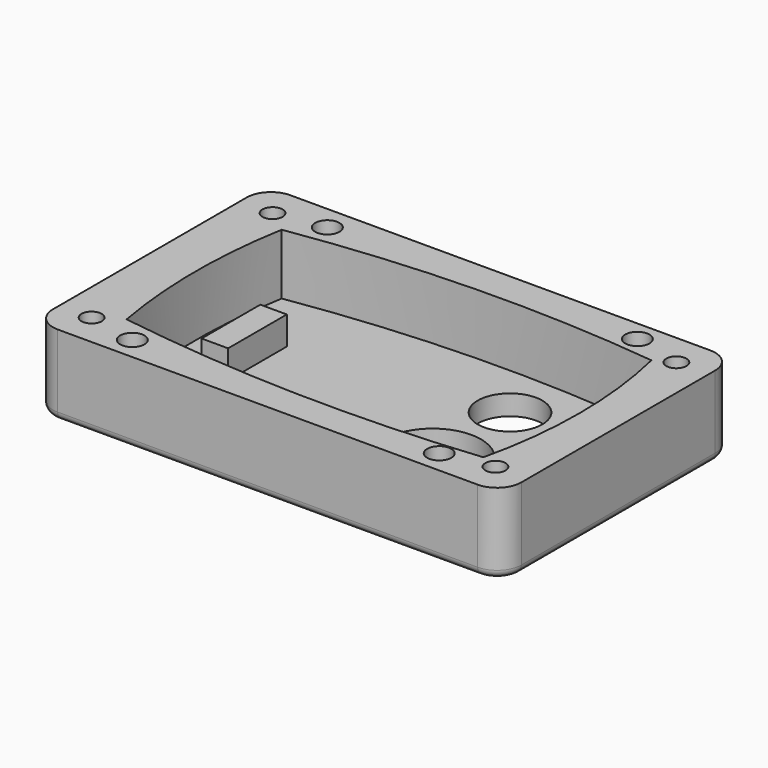
from build123d import *

# Parameters (mm, degrees)
F0_W     = 58
F0_H     = 36
F0_R     = 1.25
F0_R_2   = 1.5
F1_DEPTH = 10
F0_R_3   = 1
F0_W_2   = 3.2825097442
F0_H_2   = 9.0816104785
F0_R_4   = 4
F2_DEPTH = 2.5
F3_R     = 3
F4_DEPTH = 6
F5_START = 0.9
F5_DEPTH = 16.2
F6_START = 6
F6_DEPTH = 10.7
F7_R     = 1


with BuildPart() as f1:
    # F0 (on Top) → F1 (new body)
    with BuildSketch(Plane.XY):
        with Locations((22.1260370687, 12.181818096)):
            Rectangle(F0_W, F0_H)
        with Locations((-2.8739629313, -1.818181904)):
            Circle(F0_R, mode=Mode.SUBTRACT)
        with Locations((3.1260370687, -3.018181904)):
            Circle(F0_R_2, mode=Mode.SUBTRACT)
        with Locations((41.1260370687, -3.018181904)):
            Circle(F0_R_2, mode=Mode.SUBTRACT)
        with Locations((47.1260370687, -1.818181904)):
            Circle(F0_R, mode=Mode.SUBTRACT)
        with BuildLine():
            Line((-0.0042433119, 0.0237876128), (-0.0123524841, 0.02397218))
            Line((-0.0123524841, 0.02397218), (-0.0123524841, 0.0693824727))
            ThreePointArc((-0.0123524841, 0.0693824727), (-1.0671188126, 12.0466773263), (-0.0123524841, 24.02397218))
            ThreePointArc((-0.0123524841, 24.02397218), (22.4498159336, 26.0118318189), (44.9770614896, 25))
            ThreePointArc((44.9770614896, 25), (46.474513746, 12), (44.9770614896, -1))
            ThreePointArc((44.9770614896, -1), (22.4574664967, -1.8971785964), (0, 0))
            ThreePointArc((0, 0), (-0.0021227043, 0.0118936194), (-0.0042433119, 0.0237876128))
        make_face(mode=Mode.SUBTRACT)
        with Locations((-2.8739629313, 26.181818096)):
            Circle(F0_R, mode=Mode.SUBTRACT)
        with Locations((3.1260370687, 27.16396598)):
            Circle(F0_R_2, mode=Mode.SUBTRACT)
        with Locations((41.1260370687, 27.6376707083)):
            Circle(F0_R_2, mode=Mode.SUBTRACT)
        with Locations((47.1260370687, 26.181818096)):
            Circle(F0_R, mode=Mode.SUBTRACT)
        with Locations((-2.8739629313, 26.181818096)):
            Circle(F0_R)
        with Locations((47.1260370687, 26.181818096)):
            Circle(F0_R)
        with Locations((47.1260370687, -1.818181904)):
            Circle(F0_R)
        with Locations((-2.8739629313, -1.818181904)):
            Circle(F0_R)
        with Locations((3.1260370687, -3.018181904)):
            Circle(F0_R_2)
        with Locations((3.1260370687, 27.16396598)):
            Circle(F0_R_2)
        with Locations((41.1260370687, 27.6376707083)):
            Circle(F0_R_2)
        with Locations((41.1260370687, -3.018181904)):
            Circle(F0_R_2)
    extrude(amount=F1_DEPTH)

    # F0 (on Top) → F2 (join)
    with BuildSketch(Plane.XY):
        with BuildLine():
            ThreePointArc((-0.0123524841, 24.02397218), (-1.0671188126, 12.0466773263), (-0.0123524841, 0.0693824727))
            Line((-0.0123524841, 0.0693824727), (-0.0123524841, 24.02397218))
        make_face()
        with BuildLine():
            Line((-0.0123524841, 24.02397218), (-0.0123524841, 0.0693824727))
            ThreePointArc((-0.0123524841, 0.0693824727), (-0.0083017494, 0.0465843578), (-0.0042433119, 0.0237876128))
            Line((-0.0042433119, 0.0237876128), (44.9770614896, -1))
            Line((44.9770614896, -1), (44.9770614896, 25))
            Line((44.9770614896, 25), (-0.0123524841, 24.02397218))
        make_face()
        with Locations((2.9621722015, 2.0848012064)):
            Circle(F0_R_3, mode=Mode.SUBTRACT)
        with Locations((5.0146379508, 11.9371688925)):
            Rectangle(F0_W_2, F0_H_2, mode=Mode.SUBTRACT)
        with Locations((41.7125664489, 2.0848012064)):
            Circle(F0_R_3, mode=Mode.SUBTRACT)
        with BuildLine():
            Line((26.1260370687, 7.1930042468), (26.1260370687, 9.181818096))
            Line((26.1260370687, 9.181818096), (26.4652403515, 9.181818096))
            ThreePointArc((26.4652403515, 9.181818096), (32.1260370687, 13.1930042468), (37.7868337859, 9.181818096))
            Line((37.7868337859, 9.181818096), (38.1260370687, 9.181818096))
            Line((38.1260370687, 9.181818096), (38.1260370687, 7.1930042468))
            Line((38.1260370687, 7.1930042468), (38.1260370687, 1.181818096))
            Line((38.1260370687, 1.181818096), (26.1260370687, 1.181818096))
            Line((26.1260370687, 1.181818096), (26.1260370687, 7.1930042468))
        make_face(mode=Mode.SUBTRACT)
        with Locations((41.1260370687, 12.181818096)):
            Circle(F0_R_2, mode=Mode.SUBTRACT)
        with Locations((18.8074270263, 12.2937392443)):
            Circle(F0_R_3, mode=Mode.SUBTRACT)
        with Locations((2.9621722015, 21.6664075851)):
            Circle(F0_R_3, mode=Mode.SUBTRACT)
        with Locations((26.8074270263, 12.2937392443)):
            Circle(F0_R_3, mode=Mode.SUBTRACT)
        with Locations((32.1260370687, 19.181818096)):
            Circle(F0_R_4, mode=Mode.SUBTRACT)
        with Locations((41.7125664489, 21.6664075851)):
            Circle(F0_R_3, mode=Mode.SUBTRACT)
        with BuildLine():
            Line((44.9770614896, -1), (-0.0042433119, 0.0237876128))
            ThreePointArc((-0.0042433119, 0.0237876128), (-0.0021227043, 0.0118936194), (0, 0))
            ThreePointArc((0, 0), (22.4574664967, -1.8971785964), (44.9770614896, -1))
        make_face()
        with BuildLine():
            ThreePointArc((44.9770614896, 25), (22.4498159336, 26.0118318189), (-0.0123524841, 24.02397218))
            Line((-0.0123524841, 24.02397218), (44.9770614896, 25))
        make_face()
        with BuildLine():
            Line((44.9770614896, 25), (44.9770614896, -1))
            ThreePointArc((44.9770614896, -1), (46.474513746, 12), (44.9770614896, 25))
        make_face()
        with Locations((2.9621722015, 21.6664075851)):
            Circle(F0_R_3)
        with Locations((2.9621722015, 2.0848012064)):
            Circle(F0_R_3)
        with Locations((41.7125664489, 2.0848012064)):
            Circle(F0_R_3)
        with Locations((41.7125664489, 21.6664075851)):
            Circle(F0_R_3)
        with Locations((18.8074270263, 12.2937392443)):
            Circle(F0_R_3)
        with Locations((26.8074270263, 12.2937392443)):
            Circle(F0_R_3)
        with Locations((5.0146379508, 11.9371688925)):
            Rectangle(F0_W_2, F0_H_2)
        with BuildLine():
            Line((26.4652403515, 9.181818096), (26.1260370687, 9.181818096))
            Line((26.1260370687, 9.181818096), (26.1260370687, 7.1930042468))
            ThreePointArc((26.1260370687, 7.1930042468), (26.2114457767, 8.2017707453), (26.4652403515, 9.181818096))
        make_face()
        with BuildLine():
            ThreePointArc((38.1260370687, 7.1930042468), (32.1260370687, 1.1930042468), (26.1260370687, 7.1930042468))
            Line((26.1260370687, 7.1930042468), (26.1260370687, 1.181818096))
            Line((26.1260370687, 1.181818096), (38.1260370687, 1.181818096))
            Line((38.1260370687, 1.181818096), (38.1260370687, 7.1930042468))
        make_face()
        with BuildLine():
            Line((38.1260370687, 9.181818096), (37.7868337859, 9.181818096))
            ThreePointArc((37.7868337859, 9.181818096), (38.0406283607, 8.2017707453), (38.1260370687, 7.1930042468))
            Line((38.1260370687, 7.1930042468), (38.1260370687, 9.181818096))
        make_face()
    extrude(amount=F2_DEPTH)

    # F3
    f3_edges = [f1.edges().sort_by_distance(p)[0] for p in [
        (51.126037, 30.181818, 5),
        (51.126037, -5.818182, 5),
        (-6.873963, -5.818182, 5),
        (-6.873963, 30.181818, 5),
    ]]
    fillet(f3_edges, radius=F3_R)

    # F0 (on Top) → F4 (join)
    with BuildSketch(Plane.XY):
        with Locations((5.0146379508, 11.9371688925)):
            Rectangle(F0_W_2, F0_H_2)
    extrude(amount=F4_DEPTH)

    # F0 (on Top) → F5 (cut)
    with BuildSketch(Plane.XY.offset(F5_START)):
        with Locations((47.1260370687, 26.181818096)):
            Circle(F0_R)
        with Locations((-2.8739629313, 26.181818096)):
            Circle(F0_R)
        with Locations((-2.8739629313, -1.818181904)):
            Circle(F0_R)
        with Locations((47.1260370687, -1.818181904)):
            Circle(F0_R)
    extrude(amount=F5_DEPTH, mode=Mode.SUBTRACT)

    # F0 (on Top) → F6 (cut)
    with BuildSketch(Plane.XY.offset(F6_START)):
        with Locations((3.1260370687, 27.16396598)):
            Circle(F0_R_2)
        with Locations((41.1260370687, 27.6376707083)):
            Circle(F0_R_2)
        with Locations((41.1260370687, -3.018181904)):
            Circle(F0_R_2)
        with Locations((3.1260370687, -3.018181904)):
            Circle(F0_R_2)
    extrude(amount=F6_DEPTH, mode=Mode.SUBTRACT)

    # F7
    f7_edges = [f1.edges().sort_by_distance(p)[0] for p in [
        (51.126037, 12.181818, 0),
        (22.126037, -5.818182, 0),
        (50.247357, -4.939502, 0),
        (50.247357, 29.303138, 0),
        (22.126037, 30.181818, 0),
        (-5.995283, 29.303138, 0),
        (-6.873963, 12.181818, 0),
        (-5.995283, -4.939502, 0),
    ]]
    fillet(f7_edges, radius=F7_R)


solid = f1.part
